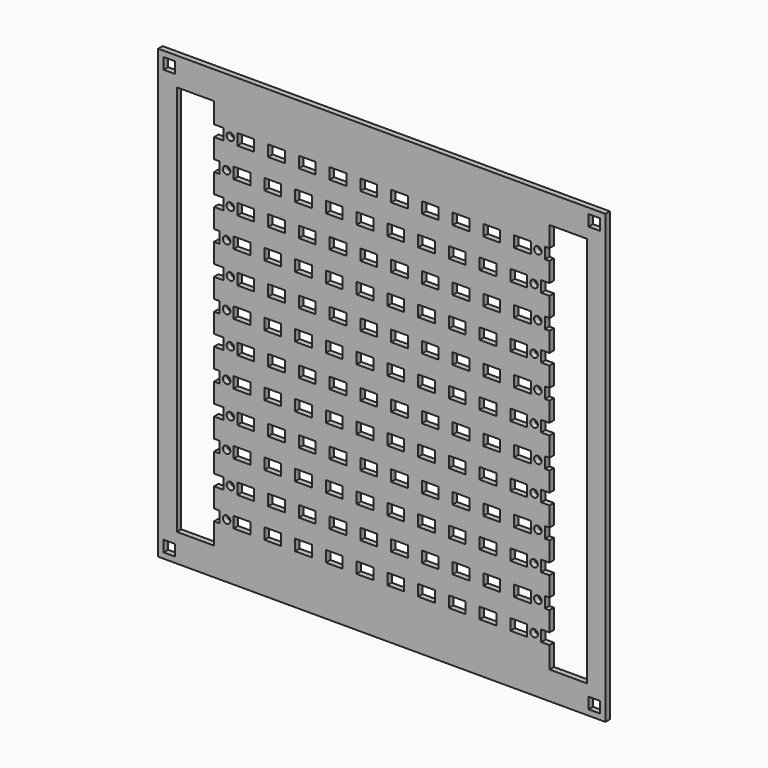
from build123d import *

# Parameters (mm, degrees)
F0_W     = 240
F0_H     = 240
F0_W_2   = 9
F0_H_2   = 6
F1_DEPTH = 3
F2_W     = 6
F2_H     = 6
F3_DEPTH = 3.001
F5_DEPTH = 3.001
F6_R     = 2
F7_DEPTH = 3.001


with BuildPart() as f1:
    # F0 (on Front) → F1 (new body)
    with BuildSketch(Plane.XZ):
        with Locations((-1.7883066535, 37.7417517798)):
            Rectangle(F0_W, F0_H)
        with Locations((-93.2883066535, -52.7582482202)):
            Rectangle(F0_W_2, F0_H_2, mode=Mode.SUBTRACT)
        with Locations((-76.7883066535, -52.7582482202)):
            Rectangle(F0_W_2, F0_H_2, mode=Mode.SUBTRACT)
        with Locations((-91.2883066535, -36.2582482202)):
            Rectangle(F0_W_2, F0_H_2, mode=Mode.SUBTRACT)
        with Locations((-74.7883066535, -36.2582482202)):
            Rectangle(F0_W_2, F0_H_2, mode=Mode.SUBTRACT)
        with Locations((-60.2883066535, -52.7582482202)):
            Rectangle(F0_W_2, F0_H_2, mode=Mode.SUBTRACT)
        with Locations((-43.7883066535, -52.7582482202)):
            Rectangle(F0_W_2, F0_H_2, mode=Mode.SUBTRACT)
        with Locations((-27.2883066535, -52.7582482202)):
            Rectangle(F0_W_2, F0_H_2, mode=Mode.SUBTRACT)
        with Locations((-10.7883066535, -52.7582482202)):
            Rectangle(F0_W_2, F0_H_2, mode=Mode.SUBTRACT)
        with Locations((-58.2883066535, -36.2582482202)):
            Rectangle(F0_W_2, F0_H_2, mode=Mode.SUBTRACT)
        with Locations((-41.7883066535, -36.2582482202)):
            Rectangle(F0_W_2, F0_H_2, mode=Mode.SUBTRACT)
        with Locations((-25.2883066535, -36.2582482202)):
            Rectangle(F0_W_2, F0_H_2, mode=Mode.SUBTRACT)
        with Locations((-8.7883066535, -36.2582482202)):
            Rectangle(F0_W_2, F0_H_2, mode=Mode.SUBTRACT)
        with Locations((-93.2883066535, -19.7582482202)):
            Rectangle(F0_W_2, F0_H_2, mode=Mode.SUBTRACT)
        with Locations((-76.7883066535, -19.7582482202)):
            Rectangle(F0_W_2, F0_H_2, mode=Mode.SUBTRACT)
        with Locations((-91.2883066535, -3.2582482202)):
            Rectangle(F0_W_2, F0_H_2, mode=Mode.SUBTRACT)
        with Locations((-74.7883066535, -3.2582482202)):
            Rectangle(F0_W_2, F0_H_2, mode=Mode.SUBTRACT)
        with Locations((-93.2883066535, 13.2417517798)):
            Rectangle(F0_W_2, F0_H_2, mode=Mode.SUBTRACT)
        with Locations((-76.7883066535, 13.2417517798)):
            Rectangle(F0_W_2, F0_H_2, mode=Mode.SUBTRACT)
        with Locations((-91.2883066535, 29.7417517798)):
            Rectangle(F0_W_2, F0_H_2, mode=Mode.SUBTRACT)
        with Locations((-74.7883066535, 29.7417517798)):
            Rectangle(F0_W_2, F0_H_2, mode=Mode.SUBTRACT)
        with Locations((-60.2883066535, -19.7582482202)):
            Rectangle(F0_W_2, F0_H_2, mode=Mode.SUBTRACT)
        with Locations((-43.7883066535, -19.7582482202)):
            Rectangle(F0_W_2, F0_H_2, mode=Mode.SUBTRACT)
        with Locations((-58.2883066535, -3.2582482202)):
            Rectangle(F0_W_2, F0_H_2, mode=Mode.SUBTRACT)
        with Locations((-41.7883066535, -3.2582482202)):
            Rectangle(F0_W_2, F0_H_2, mode=Mode.SUBTRACT)
        with Locations((-27.2883066535, -19.7582482202)):
            Rectangle(F0_W_2, F0_H_2, mode=Mode.SUBTRACT)
        with Locations((-10.7883066535, -19.7582482202)):
            Rectangle(F0_W_2, F0_H_2, mode=Mode.SUBTRACT)
        with Locations((-25.2883066535, -3.2582482202)):
            Rectangle(F0_W_2, F0_H_2, mode=Mode.SUBTRACT)
        with Locations((-8.7883066535, -3.2582482202)):
            Rectangle(F0_W_2, F0_H_2, mode=Mode.SUBTRACT)
        with Locations((-60.2883066535, 13.2417517798)):
            Rectangle(F0_W_2, F0_H_2, mode=Mode.SUBTRACT)
        with Locations((-43.7883066535, 13.2417517798)):
            Rectangle(F0_W_2, F0_H_2, mode=Mode.SUBTRACT)
        with Locations((-58.2883066535, 29.7417517798)):
            Rectangle(F0_W_2, F0_H_2, mode=Mode.SUBTRACT)
        with Locations((-41.7883066535, 29.7417517798)):
            Rectangle(F0_W_2, F0_H_2, mode=Mode.SUBTRACT)
        with Locations((-27.2883066535, 13.2417517798)):
            Rectangle(F0_W_2, F0_H_2, mode=Mode.SUBTRACT)
        with Locations((-10.7883066535, 13.2417517798)):
            Rectangle(F0_W_2, F0_H_2, mode=Mode.SUBTRACT)
        with Locations((-25.2883066535, 29.7417517798)):
            Rectangle(F0_W_2, F0_H_2, mode=Mode.SUBTRACT)
        with Locations((-8.7883066535, 29.7417517798)):
            Rectangle(F0_W_2, F0_H_2, mode=Mode.SUBTRACT)
        with Locations((5.7116933465, -52.7582482202)):
            Rectangle(F0_W_2, F0_H_2, mode=Mode.SUBTRACT)
        with Locations((22.2116933465, -52.7582482202)):
            Rectangle(F0_W_2, F0_H_2, mode=Mode.SUBTRACT)
        with Locations((38.7116933465, -52.7582482202)):
            Rectangle(F0_W_2, F0_H_2, mode=Mode.SUBTRACT)
        with Locations((55.2116933465, -52.7582482202)):
            Rectangle(F0_W_2, F0_H_2, mode=Mode.SUBTRACT)
        with Locations((7.7116933465, -36.2582482202)):
            Rectangle(F0_W_2, F0_H_2, mode=Mode.SUBTRACT)
        with Locations((24.2116933465, -36.2582482202)):
            Rectangle(F0_W_2, F0_H_2, mode=Mode.SUBTRACT)
        with Locations((40.7116933465, -36.2582482202)):
            Rectangle(F0_W_2, F0_H_2, mode=Mode.SUBTRACT)
        with Locations((57.2116933465, -36.2582482202)):
            Rectangle(F0_W_2, F0_H_2, mode=Mode.SUBTRACT)
        with Locations((71.7116933465, -52.7582482202)):
            Rectangle(F0_W_2, F0_H_2, mode=Mode.SUBTRACT)
        with Locations((88.2116933465, -52.7582482202)):
            Rectangle(F0_W_2, F0_H_2, mode=Mode.SUBTRACT)
        with Locations((73.7116933465, -36.2582482202)):
            Rectangle(F0_W_2, F0_H_2, mode=Mode.SUBTRACT)
        with Locations((90.2116933465, -36.2582482202)):
            Rectangle(F0_W_2, F0_H_2, mode=Mode.SUBTRACT)
        with Locations((5.7116933465, -19.7582482202)):
            Rectangle(F0_W_2, F0_H_2, mode=Mode.SUBTRACT)
        with Locations((22.2116933465, -19.7582482202)):
            Rectangle(F0_W_2, F0_H_2, mode=Mode.SUBTRACT)
        with Locations((7.7116933465, -3.2582482202)):
            Rectangle(F0_W_2, F0_H_2, mode=Mode.SUBTRACT)
        with Locations((24.2116933465, -3.2582482202)):
            Rectangle(F0_W_2, F0_H_2, mode=Mode.SUBTRACT)
        with Locations((38.7116933465, -19.7582482202)):
            Rectangle(F0_W_2, F0_H_2, mode=Mode.SUBTRACT)
        with Locations((55.2116933465, -19.7582482202)):
            Rectangle(F0_W_2, F0_H_2, mode=Mode.SUBTRACT)
        with Locations((40.7116933465, -3.2582482202)):
            Rectangle(F0_W_2, F0_H_2, mode=Mode.SUBTRACT)
        with Locations((57.2116933465, -3.2582482202)):
            Rectangle(F0_W_2, F0_H_2, mode=Mode.SUBTRACT)
        with Locations((5.7116933465, 13.2417517798)):
            Rectangle(F0_W_2, F0_H_2, mode=Mode.SUBTRACT)
        with Locations((22.2116933465, 13.2417517798)):
            Rectangle(F0_W_2, F0_H_2, mode=Mode.SUBTRACT)
        with Locations((7.7116933465, 29.7417517798)):
            Rectangle(F0_W_2, F0_H_2, mode=Mode.SUBTRACT)
        with Locations((24.2116933465, 29.7417517798)):
            Rectangle(F0_W_2, F0_H_2, mode=Mode.SUBTRACT)
        with Locations((38.7116933465, 13.2417517798)):
            Rectangle(F0_W_2, F0_H_2, mode=Mode.SUBTRACT)
        with Locations((55.2116933465, 13.2417517798)):
            Rectangle(F0_W_2, F0_H_2, mode=Mode.SUBTRACT)
        with Locations((40.7116933465, 29.7417517798)):
            Rectangle(F0_W_2, F0_H_2, mode=Mode.SUBTRACT)
        with Locations((57.2116933465, 29.7417517798)):
            Rectangle(F0_W_2, F0_H_2, mode=Mode.SUBTRACT)
        with Locations((71.7116933465, -19.7582482202)):
            Rectangle(F0_W_2, F0_H_2, mode=Mode.SUBTRACT)
        with Locations((73.7116933465, -3.2582482202)):
            Rectangle(F0_W_2, F0_H_2, mode=Mode.SUBTRACT)
        with Locations((88.2116933465, -19.7582482202)):
            Rectangle(F0_W_2, F0_H_2, mode=Mode.SUBTRACT)
        with Locations((90.2116933465, -3.2582482202)):
            Rectangle(F0_W_2, F0_H_2, mode=Mode.SUBTRACT)
        with Locations((71.7116933465, 13.2417517798)):
            Rectangle(F0_W_2, F0_H_2, mode=Mode.SUBTRACT)
        with Locations((73.7116933465, 29.7417517798)):
            Rectangle(F0_W_2, F0_H_2, mode=Mode.SUBTRACT)
        with Locations((88.2116933465, 13.2417517798)):
            Rectangle(F0_W_2, F0_H_2, mode=Mode.SUBTRACT)
        with Locations((90.2116933465, 29.7417517798)):
            Rectangle(F0_W_2, F0_H_2, mode=Mode.SUBTRACT)
        with Locations((-93.2883066535, 46.2417517798)):
            Rectangle(F0_W_2, F0_H_2, mode=Mode.SUBTRACT)
        with Locations((-76.7883066535, 46.2417517798)):
            Rectangle(F0_W_2, F0_H_2, mode=Mode.SUBTRACT)
        with Locations((-91.2883066535, 62.7417517798)):
            Rectangle(F0_W_2, F0_H_2, mode=Mode.SUBTRACT)
        with Locations((-74.7883066535, 62.7417517798)):
            Rectangle(F0_W_2, F0_H_2, mode=Mode.SUBTRACT)
        with Locations((-93.2883066535, 79.2417517798)):
            Rectangle(F0_W_2, F0_H_2, mode=Mode.SUBTRACT)
        with Locations((-76.7883066535, 79.2417517798)):
            Rectangle(F0_W_2, F0_H_2, mode=Mode.SUBTRACT)
        with Locations((-91.2883066535, 95.7417517798)):
            Rectangle(F0_W_2, F0_H_2, mode=Mode.SUBTRACT)
        with Locations((-74.7883066535, 95.7417517798)):
            Rectangle(F0_W_2, F0_H_2, mode=Mode.SUBTRACT)
        with Locations((-60.2883066535, 46.2417517798)):
            Rectangle(F0_W_2, F0_H_2, mode=Mode.SUBTRACT)
        with Locations((-43.7883066535, 46.2417517798)):
            Rectangle(F0_W_2, F0_H_2, mode=Mode.SUBTRACT)
        with Locations((-58.2883066535, 62.7417517798)):
            Rectangle(F0_W_2, F0_H_2, mode=Mode.SUBTRACT)
        with Locations((-41.7883066535, 62.7417517798)):
            Rectangle(F0_W_2, F0_H_2, mode=Mode.SUBTRACT)
        with Locations((-27.2883066535, 46.2417517798)):
            Rectangle(F0_W_2, F0_H_2, mode=Mode.SUBTRACT)
        with Locations((-10.7883066535, 46.2417517798)):
            Rectangle(F0_W_2, F0_H_2, mode=Mode.SUBTRACT)
        with Locations((-25.2883066535, 62.7417517798)):
            Rectangle(F0_W_2, F0_H_2, mode=Mode.SUBTRACT)
        with Locations((-8.7883066535, 62.7417517798)):
            Rectangle(F0_W_2, F0_H_2, mode=Mode.SUBTRACT)
        with Locations((-60.2883066535, 79.2417517798)):
            Rectangle(F0_W_2, F0_H_2, mode=Mode.SUBTRACT)
        with Locations((-43.7883066535, 79.2417517798)):
            Rectangle(F0_W_2, F0_H_2, mode=Mode.SUBTRACT)
        with Locations((-58.2883066535, 95.7417517798)):
            Rectangle(F0_W_2, F0_H_2, mode=Mode.SUBTRACT)
        with Locations((-41.7883066535, 95.7417517798)):
            Rectangle(F0_W_2, F0_H_2, mode=Mode.SUBTRACT)
        with Locations((-27.2883066535, 79.2417517798)):
            Rectangle(F0_W_2, F0_H_2, mode=Mode.SUBTRACT)
        with Locations((-10.7883066535, 79.2417517798)):
            Rectangle(F0_W_2, F0_H_2, mode=Mode.SUBTRACT)
        with Locations((-25.2883066535, 95.7417517798)):
            Rectangle(F0_W_2, F0_H_2, mode=Mode.SUBTRACT)
        with Locations((-8.7883066535, 95.7417517798)):
            Rectangle(F0_W_2, F0_H_2, mode=Mode.SUBTRACT)
        with Locations((-93.2883066535, 112.2417517798)):
            Rectangle(F0_W_2, F0_H_2, mode=Mode.SUBTRACT)
        with Locations((-76.7883066535, 112.2417517798)):
            Rectangle(F0_W_2, F0_H_2, mode=Mode.SUBTRACT)
        with Locations((-91.2883066535, 128.7417517798)):
            Rectangle(F0_W_2, F0_H_2, mode=Mode.SUBTRACT)
        with Locations((-74.7883066535, 128.7417517798)):
            Rectangle(F0_W_2, F0_H_2, mode=Mode.SUBTRACT)
        with Locations((-60.2883066535, 112.2417517798)):
            Rectangle(F0_W_2, F0_H_2, mode=Mode.SUBTRACT)
        with Locations((-43.7883066535, 112.2417517798)):
            Rectangle(F0_W_2, F0_H_2, mode=Mode.SUBTRACT)
        with Locations((-27.2883066535, 112.2417517798)):
            Rectangle(F0_W_2, F0_H_2, mode=Mode.SUBTRACT)
        with Locations((-10.7883066535, 112.2417517798)):
            Rectangle(F0_W_2, F0_H_2, mode=Mode.SUBTRACT)
        with Locations((-58.2883066535, 128.7417517798)):
            Rectangle(F0_W_2, F0_H_2, mode=Mode.SUBTRACT)
        with Locations((-41.7883066535, 128.7417517798)):
            Rectangle(F0_W_2, F0_H_2, mode=Mode.SUBTRACT)
        with Locations((-25.2883066535, 128.7417517798)):
            Rectangle(F0_W_2, F0_H_2, mode=Mode.SUBTRACT)
        with Locations((-8.7883066535, 128.7417517798)):
            Rectangle(F0_W_2, F0_H_2, mode=Mode.SUBTRACT)
        with Locations((5.7116933465, 46.2417517798)):
            Rectangle(F0_W_2, F0_H_2, mode=Mode.SUBTRACT)
        with Locations((22.2116933465, 46.2417517798)):
            Rectangle(F0_W_2, F0_H_2, mode=Mode.SUBTRACT)
        with Locations((7.7116933465, 62.7417517798)):
            Rectangle(F0_W_2, F0_H_2, mode=Mode.SUBTRACT)
        with Locations((24.2116933465, 62.7417517798)):
            Rectangle(F0_W_2, F0_H_2, mode=Mode.SUBTRACT)
        with Locations((38.7116933465, 46.2417517798)):
            Rectangle(F0_W_2, F0_H_2, mode=Mode.SUBTRACT)
        with Locations((55.2116933465, 46.2417517798)):
            Rectangle(F0_W_2, F0_H_2, mode=Mode.SUBTRACT)
        with Locations((40.7116933465, 62.7417517798)):
            Rectangle(F0_W_2, F0_H_2, mode=Mode.SUBTRACT)
        with Locations((57.2116933465, 62.7417517798)):
            Rectangle(F0_W_2, F0_H_2, mode=Mode.SUBTRACT)
        with Locations((5.7116933465, 79.2417517798)):
            Rectangle(F0_W_2, F0_H_2, mode=Mode.SUBTRACT)
        with Locations((22.2116933465, 79.2417517798)):
            Rectangle(F0_W_2, F0_H_2, mode=Mode.SUBTRACT)
        with Locations((7.7116933465, 95.7417517798)):
            Rectangle(F0_W_2, F0_H_2, mode=Mode.SUBTRACT)
        with Locations((24.2116933465, 95.7417517798)):
            Rectangle(F0_W_2, F0_H_2, mode=Mode.SUBTRACT)
        with Locations((38.7116933465, 79.2417517798)):
            Rectangle(F0_W_2, F0_H_2, mode=Mode.SUBTRACT)
        with Locations((55.2116933465, 79.2417517798)):
            Rectangle(F0_W_2, F0_H_2, mode=Mode.SUBTRACT)
        with Locations((40.7116933465, 95.7417517798)):
            Rectangle(F0_W_2, F0_H_2, mode=Mode.SUBTRACT)
        with Locations((57.2116933465, 95.7417517798)):
            Rectangle(F0_W_2, F0_H_2, mode=Mode.SUBTRACT)
        with Locations((71.7116933465, 46.2417517798)):
            Rectangle(F0_W_2, F0_H_2, mode=Mode.SUBTRACT)
        with Locations((73.7116933465, 62.7417517798)):
            Rectangle(F0_W_2, F0_H_2, mode=Mode.SUBTRACT)
        with Locations((88.2116933465, 46.2417517798)):
            Rectangle(F0_W_2, F0_H_2, mode=Mode.SUBTRACT)
        with Locations((90.2116933465, 62.7417517798)):
            Rectangle(F0_W_2, F0_H_2, mode=Mode.SUBTRACT)
        with Locations((71.7116933465, 79.2417517798)):
            Rectangle(F0_W_2, F0_H_2, mode=Mode.SUBTRACT)
        with Locations((73.7116933465, 95.7417517798)):
            Rectangle(F0_W_2, F0_H_2, mode=Mode.SUBTRACT)
        with Locations((88.2116933465, 79.2417517798)):
            Rectangle(F0_W_2, F0_H_2, mode=Mode.SUBTRACT)
        with Locations((90.2116933465, 95.7417517798)):
            Rectangle(F0_W_2, F0_H_2, mode=Mode.SUBTRACT)
        with Locations((5.7116933465, 112.2417517798)):
            Rectangle(F0_W_2, F0_H_2, mode=Mode.SUBTRACT)
        with Locations((22.2116933465, 112.2417517798)):
            Rectangle(F0_W_2, F0_H_2, mode=Mode.SUBTRACT)
        with Locations((38.7116933465, 112.2417517798)):
            Rectangle(F0_W_2, F0_H_2, mode=Mode.SUBTRACT)
        with Locations((55.2116933465, 112.2417517798)):
            Rectangle(F0_W_2, F0_H_2, mode=Mode.SUBTRACT)
        with Locations((7.7116933465, 128.7417517798)):
            Rectangle(F0_W_2, F0_H_2, mode=Mode.SUBTRACT)
        with Locations((24.2116933465, 128.7417517798)):
            Rectangle(F0_W_2, F0_H_2, mode=Mode.SUBTRACT)
        with Locations((40.7116933465, 128.7417517798)):
            Rectangle(F0_W_2, F0_H_2, mode=Mode.SUBTRACT)
        with Locations((57.2116933465, 128.7417517798)):
            Rectangle(F0_W_2, F0_H_2, mode=Mode.SUBTRACT)
        with Locations((71.7116933465, 112.2417517798)):
            Rectangle(F0_W_2, F0_H_2, mode=Mode.SUBTRACT)
        with Locations((88.2116933465, 112.2417517798)):
            Rectangle(F0_W_2, F0_H_2, mode=Mode.SUBTRACT)
        with Locations((73.7116933465, 128.7417517798)):
            Rectangle(F0_W_2, F0_H_2, mode=Mode.SUBTRACT)
        with Locations((90.2116933465, 128.7417517798)):
            Rectangle(F0_W_2, F0_H_2, mode=Mode.SUBTRACT)
    extrude(amount=F1_DEPTH)

    # F2 (on face) → F3 (cut, through all)
    with BuildSketch(Plane.XZ.offset(3)):
        with Locations((-115.7883066535, 151.7417517798)):
            Rectangle(F2_W, F2_H)
        with Locations((112.2116933465, 151.7417517798)):
            Rectangle(F2_W, F2_H)
        with Locations((112.2116933465, -76.2582482202)):
            Rectangle(F2_W, F2_H)
        with Locations((-115.7883066535, -76.2582482202)):
            Rectangle(F2_W, F2_H)
    extrude(amount=-F3_DEPTH, mode=Mode.SUBTRACT)

    # F4 (on face) → F5 (cut, through all)
    with BuildSketch(Plane.XZ.offset(3)):
        Polygon((-91.7883066535, 142.7417517798), (-111.7883066535, 142.7417517798), (-111.7883066535, -67.2582482202), (-91.7883066535, -67.2582482202), (-91.7883066535, -55.7582482202), (-97.7883066535, -55.7582482202), (-97.7883066535, -49.7582482202), (-91.7883066535, -49.7582482202), (-91.7883066535, -39.2582482202), (-95.7883066535, -39.2582482202), (-95.7883066535, -33.2582482202), (-91.7883066535, -33.2582482202), (-91.7883066535, -22.7582482202), (-97.7883066535, -22.7582482202), (-97.7883066535, -16.7582482202), (-91.7883066535, -16.7582482202), (-91.7883066535, -6.2582482202), (-95.7883066535, -6.2582482202), (-95.7883066535, -0.2582482202), (-91.7883066535, -0.2582482202), (-91.7883066535, 10.2417517798), (-97.7883066535, 10.2417517798), (-97.7883066535, 16.2417517798), (-91.7883066535, 16.2417517798), (-91.7883066535, 26.7417517798), (-95.7883066535, 26.7417517798), (-95.7883066535, 32.7417517798), (-91.7883066535, 32.7417517798), (-91.7883066535, 43.2417517798), (-97.7883066535, 43.2417517798), (-97.7883066535, 49.2417517798), (-91.7883066535, 49.2417517798), (-91.7883066535, 59.7417517798), (-95.7883066535, 59.7417517798), (-95.7883066535, 65.7417517798), (-91.7883066535, 65.7417517798), (-91.7883066535, 76.2417517798), (-97.7883066535, 76.2417517798), (-97.7883066535, 82.2417517798), (-91.7883066535, 82.2417517798), (-91.7883066535, 92.7417517798), (-95.7883066535, 92.7417517798), (-95.7883066535, 98.7417517798), (-91.7883066535, 98.7417517798), (-91.7883066535, 109.2417517798), (-97.7883066535, 109.2417517798), (-97.7883066535, 115.2417517798), (-91.7883066535, 115.2417517798), (-91.7883066535, 125.7417517798), (-95.7883066535, 125.7417517798), (-95.7883066535, 131.7417517798), (-91.7883066535, 131.7417517798), align=None)
        Polygon((88.2116933465, -67.2582482202), (108.2116933465, -67.2582482202), (108.2116933465, 142.7417517798), (88.2116933465, 142.7417517798), (88.2116933465, 131.7417517798), (94.7116933465, 131.7417517798), (94.7116933465, 125.7417517798), (88.2116933465, 125.7417517798), (88.2116933465, 115.2417517798), (92.7116933465, 115.2417517798), (92.7116933465, 109.2417517798), (88.2116933465, 109.2417517798), (88.2116933465, 98.7417517798), (94.7116933465, 98.7417517798), (94.7116933465, 92.7417517798), (88.2116933465, 92.7417517798), (88.2116933465, 82.2417517798), (92.7116933465, 82.2417517798), (92.7116933465, 76.2417517798), (88.2116933465, 76.2417517798), (88.2116933465, 65.7417517798), (94.7116933465, 65.7417517798), (94.7116933465, 59.7417517798), (88.2116933465, 59.7417517798), (88.2116933465, 49.2417517798), (92.7116933465, 49.2417517798), (92.7116933465, 43.2417517798), (88.2116933465, 43.2417517798), (88.2116933465, 32.7417517798), (94.7116933465, 32.7417517798), (94.7116933465, 26.7417517798), (88.2116933465, 26.7417517798), (88.2116933465, 16.2417517798), (92.7116933465, 16.2417517798), (92.7116933465, 10.2417517798), (88.2116933465, 10.2417517798), (88.2116933465, -0.2582482202), (94.7116933465, -0.2582482202), (94.7116933465, -6.2582482202), (88.2116933465, -6.2582482202), (88.2116933465, -16.7582482202), (92.7116933465, -16.7582482202), (92.7116933465, -22.7582482202), (88.2116933465, -22.7582482202), (88.2116933465, -33.2582482202), (94.7116933465, -33.2582482202), (94.7116933465, -39.2582482202), (88.2116933465, -39.2582482202), (88.2116933465, -49.7582482202), (92.7116933465, -49.7582482202), (92.7116933465, -55.7582482202), (88.2116933465, -55.7582482202), align=None)
    extrude(amount=-F5_DEPTH, mode=Mode.SUBTRACT)

    # F6 (on face) → F7 (cut, through all)
    with BuildSketch(Plane.XZ.offset(3)):
        with BuildLine():
            ThreePointArc((-83.0383066535, 112.2417517798), (-85.0383066535, 114.2417517798), (-87.0383066535, 112.2417517798))
            Line((-87.0383066535, 112.2417517798), (-83.0383066535, 112.2417517798))
        make_face()
        with BuildLine():
            Line((-83.0383066535, 112.2417517798), (-87.0383066535, 112.2417517798))
            ThreePointArc((-87.0383066535, 112.2417517798), (-85.0383066535, 110.2417517798), (-83.0383066535, 112.2417517798))
        make_face()
        with BuildLine():
            ThreePointArc((-81.0383066535, 128.7417517798), (-83.0383066535, 130.7417517798), (-85.0383066535, 128.7417517798))
            Line((-85.0383066535, 128.7417517798), (-81.0383066535, 128.7417517798))
        make_face()
        with BuildLine():
            Line((-81.0383066535, 128.7417517798), (-85.0383066535, 128.7417517798))
            ThreePointArc((-85.0383066535, 128.7417517798), (-83.0383066535, 126.7417517798), (-81.0383066535, 128.7417517798))
        make_face()
        with Locations((-83.0383066535, 95.7417517798)):
            Circle(F6_R)
        with Locations((-85.0383066535, 79.2417517798)):
            Circle(F6_R)
        with Locations((-83.0383066535, 62.7417517798)):
            Circle(F6_R)
        with Locations((-85.0383066535, 46.2417517798)):
            Circle(F6_R)
        with Locations((-83.0383066535, 29.7417517798)):
            Circle(F6_R)
        with Locations((-85.0383066535, 13.2417517798)):
            Circle(F6_R)
        with Locations((-83.0383066535, -3.2582482202)):
            Circle(F6_R)
        with Locations((-85.0383066535, -19.7582482202)):
            Circle(F6_R)
        with Locations((-83.0383066535, -36.2582482202)):
            Circle(F6_R)
        with Locations((-85.0383066535, -52.7582482202)):
            Circle(F6_R)
        with BuildLine():
            ThreePointArc((83.9616933465, 128.7417517798), (81.9616933465, 130.7417517798), (79.9616933465, 128.7417517798))
            Line((79.9616933465, 128.7417517798), (83.9616933465, 128.7417517798))
        make_face()
        with BuildLine():
            Line((83.9616933465, 128.7417517798), (79.9616933465, 128.7417517798))
            ThreePointArc((79.9616933465, 128.7417517798), (81.9616933465, 126.7417517798), (83.9616933465, 128.7417517798))
        make_face()
        with BuildLine():
            ThreePointArc((81.9616933465, 112.2417517798), (79.9616933465, 114.2417517798), (77.9616933465, 112.2417517798))
            Line((77.9616933465, 112.2417517798), (81.9616933465, 112.2417517798))
        make_face()
        with BuildLine():
            Line((81.9616933465, 112.2417517798), (77.9616933465, 112.2417517798))
            ThreePointArc((77.9616933465, 112.2417517798), (79.9616933465, 110.2417517798), (81.9616933465, 112.2417517798))
        make_face()
        with Locations((81.9616933465, 95.7417517798)):
            Circle(F6_R)
        with Locations((79.9616933465, 79.2417517798)):
            Circle(F6_R)
        with Locations((81.9616933465, 62.7417517798)):
            Circle(F6_R)
        with Locations((79.9616933465, 46.2417517798)):
            Circle(F6_R)
        with Locations((81.9616933465, 29.7417517798)):
            Circle(F6_R)
        with Locations((79.9616933465, 13.2417517798)):
            Circle(F6_R)
        with Locations((81.9616933465, -3.2582482202)):
            Circle(F6_R)
        with Locations((79.9616933465, -19.7582482202)):
            Circle(F6_R)
        with Locations((81.9616933465, -36.2582482202)):
            Circle(F6_R)
        with Locations((79.9616933465, -52.7582482202)):
            Circle(F6_R)
    extrude(amount=-F7_DEPTH, mode=Mode.SUBTRACT)


solid = f1.part
